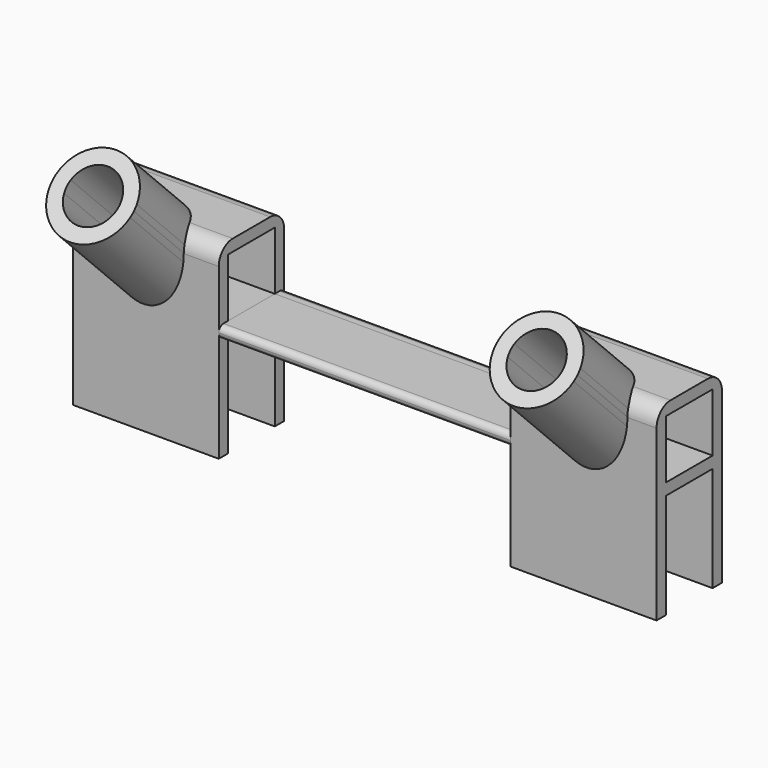
from build123d import *

# Parameters (mm, degrees)
F1_DEPTH      = 25
F2_ANGLE      = 45
F3_W          = 2
F3_H          = 18
F4_DEPTH      = 50
F4_DEPTH_BACK = 50
F5_DEPTH      = 25
F5_DEPTH_BACK = 25
F6_DEPTH      = 25
F6_DEPTH_BACK = 25
F3_W_2        = 10
F3_H_2        = 10
F7_DEPTH      = 50
F7_DEPTH_BACK = 50
F8_R          = 3
F9_R          = 0.99999


# Not quite as in the source:
# - a fillet or chamfer is up to 0.001 mm smaller than in the source, because OpenCascade refuses the exact size


with BuildPart() as f1:
    # F0 (on Front) → F1 (new body)
    with BuildSketch(Plane.XZ):
        with BuildLine():
            Line((-33.6125178063, 23.0619773716), (-31.0717967697, 23.0619773716))
            ThreePointArc((-31.0717967697, 23.0619773716), (-38, 29.0619773716), (-44.9282032303, 23.0619773716))
            Line((-44.9282032303, 23.0619773716), (-42.3874821937, 23.0619773716))
            ThreePointArc((-42.3874821937, 23.0619773716), (-38, 26.5619773716), (-33.6125178063, 23.0619773716))
        make_face()
        with BuildLine():
            Line((-42.3874821937, 23.0619773716), (-44.9282032303, 23.0619773716))
            ThreePointArc((-44.9282032303, 23.0619773716), (-45, 22.0619773716), (-44.9282032303, 21.0619773716))
            Line((-44.9282032303, 21.0619773716), (-42.3874821937, 21.0619773716))
            ThreePointArc((-42.3874821937, 21.0619773716), (-42.5, 22.0619773716), (-42.3874821937, 23.0619773716))
        make_face()
        with BuildLine():
            ThreePointArc((-44.9282032303, 21.0619773716), (-38, 15.0619773716), (-31.0717967697, 21.0619773716))
            Line((-31.0717967697, 21.0619773716), (-33.6125178063, 21.0619773716))
            ThreePointArc((-33.6125178063, 21.0619773716), (-38, 17.5619773716), (-42.3874821937, 21.0619773716))
            Line((-42.3874821937, 21.0619773716), (-44.9282032303, 21.0619773716))
        make_face()
        with BuildLine():
            ThreePointArc((-31.0717967697, 21.0619773716), (-31.017972264, 21.560690334), (-31, 22.0619773716))
            ThreePointArc((-31, 22.0619773716), (-31.017972264, 22.5632644091), (-31.0717967697, 23.0619773716))
            Line((-31.0717967697, 23.0619773716), (-33.6125178063, 23.0619773716))
            ThreePointArc((-33.6125178063, 23.0619773716), (-33.5282179239, 22.565132481), (-33.5, 22.0619773716))
            ThreePointArc((-33.5, 22.0619773716), (-33.5282179239, 21.5588222621), (-33.6125178063, 21.0619773716))
            Line((-33.6125178063, 21.0619773716), (-31.0717967697, 21.0619773716))
        make_face()
    extrude(amount=F1_DEPTH)


with BuildPart() as f1b:
    # F0 (on Front) → F1, piece 2 (new body)
    with BuildSketch(Plane.XZ):
        with BuildLine():
            ThreePointArc((44.9282032303, 23.0619773716), (38, 29.0619773716), (31.0717967697, 23.0619773716))
            Line((31.0717967697, 23.0619773716), (33.6125178063, 23.0619773716))
            ThreePointArc((33.6125178063, 23.0619773716), (38, 26.5619773716), (42.3874821937, 23.0619773716))
            Line((42.3874821937, 23.0619773716), (44.9282032303, 23.0619773716))
        make_face()
        with BuildLine():
            Line((33.6125178063, 23.0619773716), (31.0717967697, 23.0619773716))
            ThreePointArc((31.0717967697, 23.0619773716), (31, 22.0619773716), (31.0717967697, 21.0619773716))
            Line((31.0717967697, 21.0619773716), (33.6125178063, 21.0619773716))
            ThreePointArc((33.6125178063, 21.0619773716), (33.5, 22.0619773716), (33.6125178063, 23.0619773716))
        make_face()
        with BuildLine():
            Line((33.6125178063, 21.0619773716), (31.0717967697, 21.0619773716))
            ThreePointArc((31.0717967697, 21.0619773716), (38, 15.0619773716), (44.9282032303, 21.0619773716))
            Line((44.9282032303, 21.0619773716), (42.3874821937, 21.0619773716))
            ThreePointArc((42.3874821937, 21.0619773716), (38, 17.5619773716), (33.6125178063, 21.0619773716))
        make_face()
        with BuildLine():
            ThreePointArc((45, 22.0619773716), (44.982027736, 22.5632644091), (44.9282032303, 23.0619773716))
            Line((44.9282032303, 23.0619773716), (42.3874821937, 23.0619773716))
            ThreePointArc((42.3874821937, 23.0619773716), (42.4717820761, 22.565132481), (42.5, 22.0619773716))
            ThreePointArc((42.5, 22.0619773716), (42.4717820761, 21.5588222621), (42.3874821937, 21.0619773716))
            Line((42.3874821937, 21.0619773716), (44.9282032303, 21.0619773716))
            ThreePointArc((44.9282032303, 21.0619773716), (44.982027736, 21.560690334), (45, 22.0619773716))
        make_face()
    extrude(amount=F1_DEPTH)


with BuildPart() as f1_1:
    # F2: moved
    add(f1.part.rotate(Axis((25, 0, 22.0619773716), (-1, 0, 0)), F2_ANGLE))


with BuildPart() as f1b_1:
    # F2: moved
    add(f1b.part.rotate(Axis((25, 0, 22.0619773716), (-1, 0, 0)), F2_ANGLE))


with BuildPart() as f4:
    # F3 (on Right) → F4 (new body, two sides)
    with BuildSketch(Plane.YZ) as f4_sk:
        Polygon((7, 20.0315864533), (5, 20), (-5, 20), (-7, 20), (-7, 18), (-5, 18), (5, 18), (7, 18), align=None)
        Polygon((5, 30), (5, 20), (7, 20.0315864533), (7, 32), (-7, 32), (-7, 20), (-5, 20), (-5, 30), align=None)
        with Locations((6, 9)):
            Rectangle(F3_W, F3_H)
        with Locations((-6, 9)):
            Rectangle(F3_W, F3_H)
    extrude(amount=F4_DEPTH)
    extrude(f4_sk.sketch, amount=-F4_DEPTH_BACK)

    # F3 (on Right) → F5 (cut, two sides)
    with BuildSketch(Plane.YZ) as f5_sk:
        Polygon((7, 20.0315864533), (5, 20), (-5, 20), (-7, 20), (-7, 18), (-5, 18), (5, 18), (7, 18), align=None)
        Polygon((5, 30), (5, 20), (7, 20.0315864533), (7, 32), (-7, 32), (-7, 20), (-5, 20), (-5, 30), align=None)
        with Locations((6, 9)):
            Rectangle(F3_W, F3_H)
        with Locations((-6, 9)):
            Rectangle(F3_W, F3_H)
    extrude(amount=-F5_DEPTH, mode=Mode.SUBTRACT)
    extrude(f5_sk.sketch, amount=F5_DEPTH_BACK, mode=Mode.SUBTRACT)

    # F8
    f8_edges = [f4.edges().sort_by_distance(p)[0] for p in [
        (37.5, 7, 32),
        (-37.5, 7, 32),
        (37.5, -7, 32),
        (-37.5, -7, 32),
    ]]
    fillet(f8_edges, radius=F8_R)


with BuildPart() as f6:
    # F3 (on Right) → F6 (new body, two sides)
    with BuildSketch(Plane.YZ) as f6_sk:
        Polygon((7, 20.0315864533), (5, 20), (-5, 20), (-7, 20), (-7, 18), (-5, 18), (5, 18), (7, 18), align=None)
    extrude(amount=F6_DEPTH)
    extrude(f6_sk.sketch, amount=-F6_DEPTH_BACK)

    # F9 (radius 1 in the source; OpenCascade refuses exactly that, so slightly less here)
    f9_edges = [f6.edges().sort_by_distance(p)[0] for p in [
        (0, -7, 20),
        (0, -7, 18),
        (0, 7, 20.031586),
        (0, 7, 18),
    ]]
    fillet(f9_edges, radius=F9_R)


with BuildPart() as f7_tool:
    # F3 (on Right) → F7 (new body, two sides)
    with BuildSketch(Plane.YZ) as f7_sk:
        with Locations((0, 25)):
            Rectangle(F3_W_2, F3_H_2)
    extrude(amount=-F7_DEPTH)
    extrude(f7_sk.sketch, amount=F7_DEPTH_BACK)


with BuildPart() as f1_2:
    add(f1_1.part)

    # F7: cut by f7_tool
    add(f7_tool.part, mode=Mode.SUBTRACT)


with BuildPart() as f1b_2:
    add(f1b_1.part)

    # F7: cut by f7_tool
    add(f7_tool.part, mode=Mode.SUBTRACT)


solid = Compound([f4.part, f6.part, f1_2.part, f1b_2.part])
